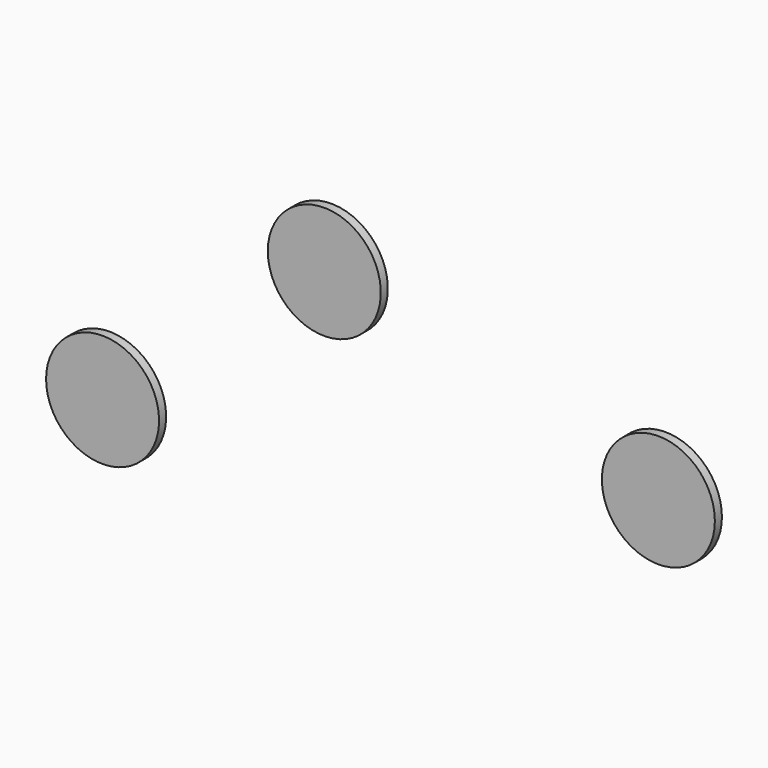
from build123d import *

# Parameters (mm, degrees)
F0_R      = 203.2
F1_DEPTH  = 15.875
F7_R      = 203.2
F8_DEPTH  = 31.75
F9_R      = 203.2
F10_DEPTH = 31.75


# Not quite as in the source:
# - the program builds the solid bodies; features that only make, move or delete a surface that nothing else refers to are left out


with BuildPart() as f1:
    # F0 (on Front) → F1 (new body, symmetric)
    with BuildSketch(Plane.XZ):
        Circle(F0_R)
    extrude(amount=F1_DEPTH, both=True)


with BuildPart() as f8:
    # F7 (on plane+point) → F8 (new body)
    with BuildSketch(Plane(origin=(0, 482.6, 0), x_dir=(-1, 0, 0), z_dir=(0, 1, 0))):
        with Locations((1600.4558962578, 0)):
            Circle(F7_R)
    extrude(amount=F8_DEPTH)


with BuildPart() as f10:
    # F9 (on plane+point) → F10 (new body)
    with BuildSketch(Plane(origin=(0, -482.6, 0), x_dir=(-1, 0, 0), z_dir=(0, 1, 0))):
        with Locations((1600.4558962578, 0)):
            Circle(F9_R)
    extrude(amount=-F10_DEPTH)


solid = Compound([f1.part, f8.part, f10.part])
